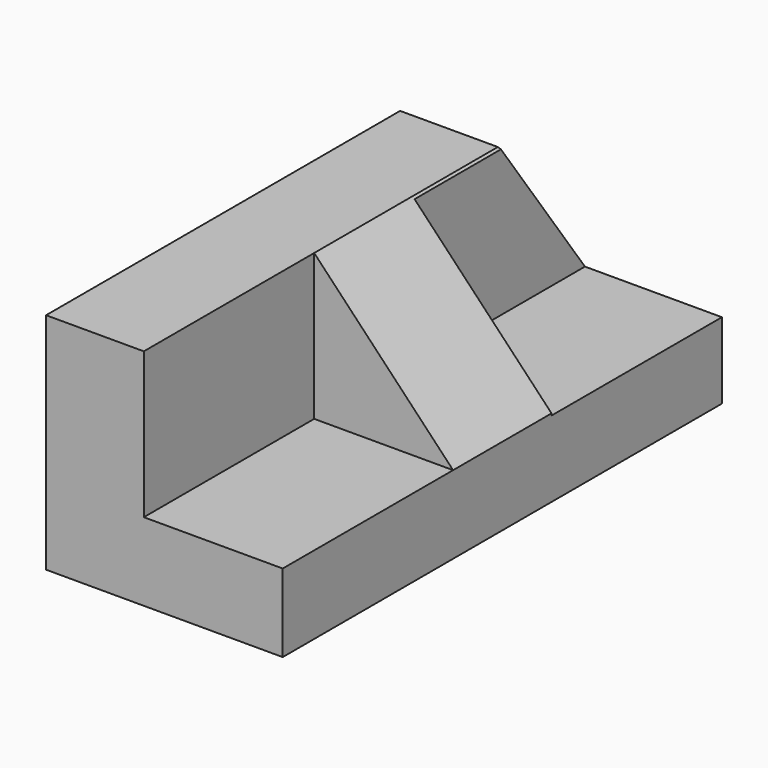
from build123d import *

# Parameters (mm, degrees)
F0_W      = 63.5
F0_H      = 36.0719883448
F1_DEPTH  = 25.4
F2_DEPTH  = 62.992
F4_W      = 47.7636682294
F4_H      = 23.5122792056
F5_DEPTH  = 34.29
F3_W      = 47.4535489879
F3_H      = 23.8223956531
F6_DEPTH  = 34.29
F8_DEPTH  = 25.4
F9_DEPTH  = 25.4
F11_DEPTH = 41.402


with BuildPart() as f1:
    # F0 (on Front) → F1 (new body)
    with BuildSketch(Plane.XZ):
        with Locations((-40.8926705517, 18.0359941724)):
            Rectangle(F0_W, F0_H)
    extrude(amount=F1_DEPTH)

    # F2 (add): a face of the model
    f2_faces = [f1.faces().sort_by_distance(p)[0] for p in [
        (-40.8926705517, 0, 18.0359941724),
    ]]
    extrude(f2_faces, amount=F2_DEPTH)

    # F4 (on face) → F5 (cut)
    with BuildSketch(Plane.XZ.offset(25.4)):
        with Locations((-33.0245046664, 24.315848742)):
            Rectangle(F4_W, F4_H)
    extrude(amount=-F5_DEPTH, mode=Mode.SUBTRACT)

    # F3 (on face) → F6 (cut)
    with BuildSketch(Plane(origin=(0, 62.992, 0), x_dir=(-1, 0, 0), z_dir=(0, 1, 0))):
        with Locations((32.8694450457, 24.1607905182)):
            Rectangle(F3_W, F3_H)
    extrude(amount=-F6_DEPTH, mode=Mode.SUBTRACT)

    # F8 (cut): a face of the model
    f8_faces = [f1.faces().sort_by_distance(p)[0] for p in [
        (-9.1426705517, 18.6122366805, 11.6054298815),
    ]]
    extrude(f8_faces, amount=-F8_DEPTH, mode=Mode.SUBTRACT)

    # F7 (on face) → F9 (cut)
    with BuildSketch(Plane.YZ.offset(-56.5962195396)):
        Polygon((62.992, 36.0719883448), (45.847, 36.0719883448), (62.992, 12.2495926917), align=None)
    extrude(amount=-F9_DEPTH, mode=Mode.SUBTRACT)

    # F10 (on face) → F11 (cut)
    with BuildSketch(Plane.XZ.offset(-8.89)):
        Polygon((-34.5426705517, 36.0719883448), (-56.9063387811, 36.0719883448), (-34.5426705517, 12.5597091392), align=None)
    extrude(amount=-F11_DEPTH, mode=Mode.SUBTRACT)


solid = f1.part
